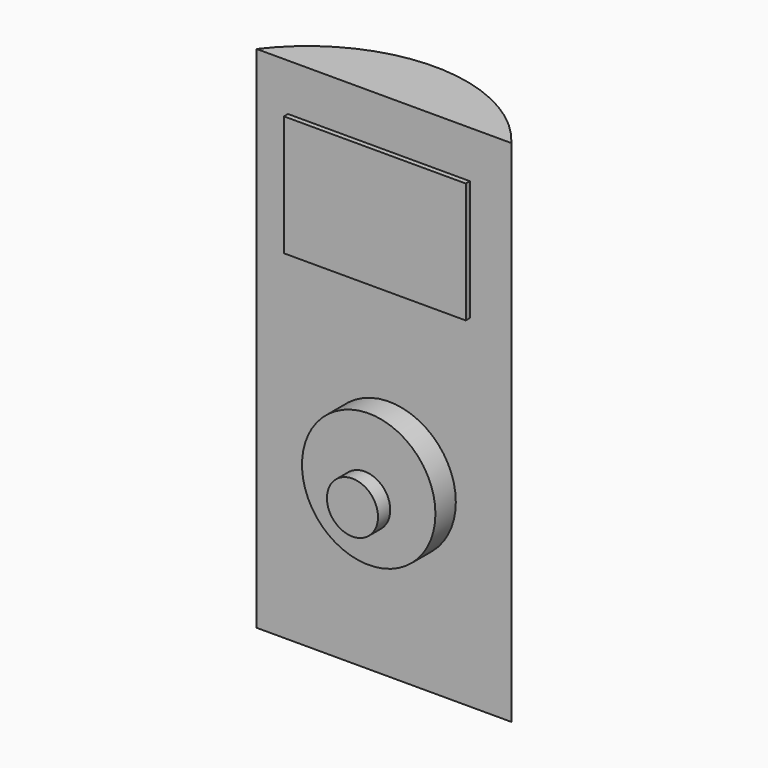
from build123d import *

# Parameters (mm, degrees)
F1_DEPTH  = 127
F2_R      = 16.6289302691
F3_DEPTH  = 6.35
F4_W      = 2.8006685898
F4_H      = 13.494130224
F4_W_2    = 2.8006681241
F4_H_2    = 14.0033438802
F5_DEPTH  = 2.54
F6_R      = 6.3651576638
F7_DEPTH  = 3.81
F10_W     = 45.3136
F10_H     = 30.0435274839
F11_DEPTH = 1.27


# Not quite as in the source:
# - a feature of the source that left no trace in its solid (it failed there, or was rolled back) is left out


with BuildPart() as f1:
    # F0 (on Top) → F1 (new body)
    with BuildSketch(Plane.XY):
        with BuildLine():
            ThreePointArc((24.3542956412, 0), (-7.3957043588, 15.8499764569), (-39.1457043588, 0))
            Line((-39.1457043588, 0), (24.3542956412, 0))
        make_face()
    extrude(amount=F1_DEPTH)

    # F2 (on face) → F3 (join)
    with BuildSketch(Plane.XZ):
        with Locations((-6.1257043588, 43.7316484749)):
            Circle(F2_R)
    extrude(amount=F3_DEPTH)

    # F4 (on face) → F5 (join)
    with BuildSketch(Plane.XZ.offset(6.35)):
        with Locations((-15.4036753811, 41.3128901273)):
            Rectangle(F4_W, F4_H)
        with Locations((1.4003340621, 41.0582832992)):
            Rectangle(F4_W_2, F4_H_2)
    extrude(amount=-F5_DEPTH)

    # F6 (on face) → F7 (join)
    with BuildSketch(Plane.XZ.offset(6.35)):
        with Locations((-7.1289734915, 40.9309826791)):
            Circle(F6_R)
    extrude(amount=F7_DEPTH)

    # F10 (on face) → F11 (join)
    with BuildSketch(Plane.XZ):
        with Locations((-8.6597625557, 100.2542302012)):
            Rectangle(F10_W, F10_H)
    extrude(amount=F11_DEPTH)


solid = f1.part
